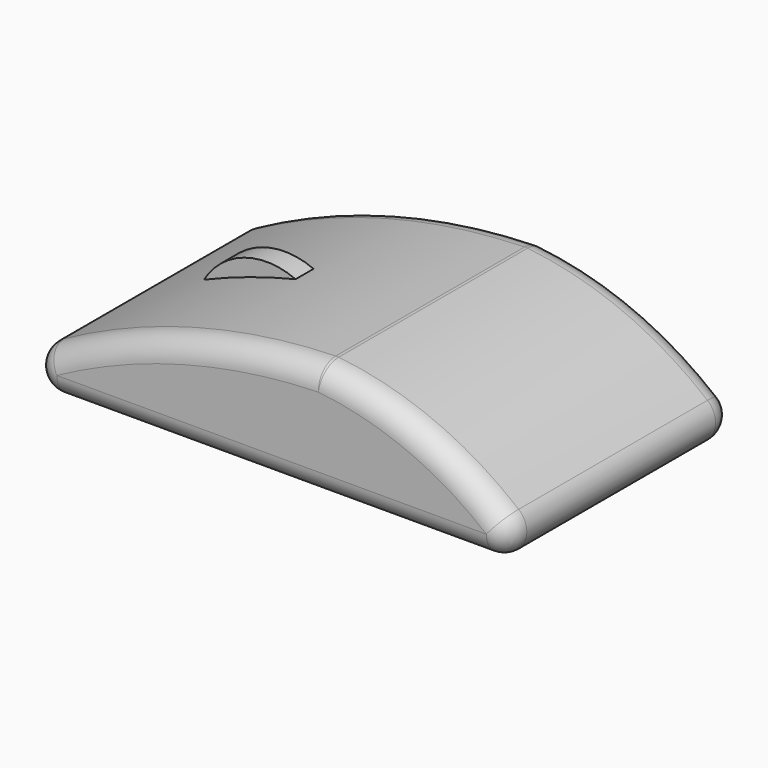
from build123d import *

# Parameters (mm, degrees)
F1_DEPTH      = 31.75
F1_DEPTH_BACK = 31.75
F2_DEPTH      = 2.54
F2_DEPTH_BACK = 2.54
F3_F1_R       = 5.08
F3_F2_R       = 5.08
F3_F3_R       = 5.08
F3_F4_R       = 5.0799
F3_F5_R       = 5.0799
F5_W          = 6.8330275826
F5_H          = 2.7183471248
F6_DEPTH      = 0.254


# Not quite as in the source:
# - a fillet or chamfer is up to 0.001 mm smaller than in the source, because OpenCascade refuses the exact size


with BuildPart() as f1:
    # F0 (on Front) → F1 (new body, two sides)
    with BuildSketch(Plane.XZ) as f1_sk:
        with BuildLine():
            ThreePointArc((-25.8951373398, -5.5155940354), (-40.0289198751, -12.4604967705), (-53.2617530078, -20.9979208572))
            Line((-53.2617530078, -20.9979208572), (73.7382469922, -20.9979208572))
            ThreePointArc((73.7382469922, -20.9979208572), (51.1172189887, -3.1620431242), (23.5122566854, 5.0717590762))
            ThreePointArc((23.5122566854, 5.0717590762), (9.0495911456, 3.953982117), (-5.2107890931, 1.2969771686))
            ThreePointArc((-5.2107890931, 1.2969771686), (-15.6900093901, -1.6932084475), (-25.8951373398, -5.5155940354))
        make_face()
    extrude(amount=F1_DEPTH)
    extrude(f1_sk.sketch, amount=-F1_DEPTH_BACK)

    # F0 (on Front) → F2 (join, two sides)
    with BuildSketch(Plane.XZ) as f2_sk:
        with BuildLine():
            ThreePointArc((-5.2107890931, 1.2969771686), (-16.8447265846, 1.8127472133), (-25.8951373398, -5.5155940354))
            ThreePointArc((-25.8951373398, -5.5155940354), (-15.6900093901, -1.6932084475), (-5.2107890931, 1.2969771686))
        make_face()
    extrude(amount=F2_DEPTH)
    extrude(f2_sk.sketch, amount=-F2_DEPTH_BACK)

    # F3: fillet of radius 5.08 on 9 edges, made by hand

    # F3_f1
    f3_f1_edges = [f1.edges().sort_by_distance(p)[0] for p in [
        (73.7382469922, 0, -20.9979208572),
    ]]
    fillet(f3_f1_edges, radius=F3_F1_R)

    # F3_f2
    f3_f2_edges = [f1.edges().sort_by_distance(p)[0] for p in [
        (23.5122566854, 0, 5.0717590762),
    ]]
    fillet(f3_f2_edges, radius=F3_F2_R)

    # F3_f3
    f3_f3_edges = [f1.edges().sort_by_distance(p)[0] for p in [
        (-53.2617530078, 0, -20.9979208572),
    ]]
    fillet(f3_f3_edges, radius=F3_F3_R)

    # F3_f4 (radius 5.08 in the source; OpenCascade refuses exactly that, so slightly less here)
    f3_f4_edges = [f1.edges().sort_by_distance(p)[0] for p in [
        (-8.5056935283, 31.75, 0.4546248012),
    ]]
    fillet(f3_f4_edges, radius=F3_F4_R)

    # F3_f5 (radius 5.08 in the source; OpenCascade refuses exactly that, so slightly less here)
    f3_f5_edges = [f1.edges().sort_by_distance(p)[0] for p in [
        (-8.5056935283, -31.75, 0.4546248012),
    ]]
    fillet(f3_f5_edges, radius=F3_F5_R)

    # F5 (on face) → F6 (join)
    with BuildSketch(Plane(origin=(0, 0, -20.9979208572), x_dir=(1, 0, 0), z_dir=(0, 0, -1))):
        with Locations((3.4165137913, -12.3521317728)):
            Rectangle(F5_W, F5_H)
    extrude(amount=F6_DEPTH)


solid = f1.part
